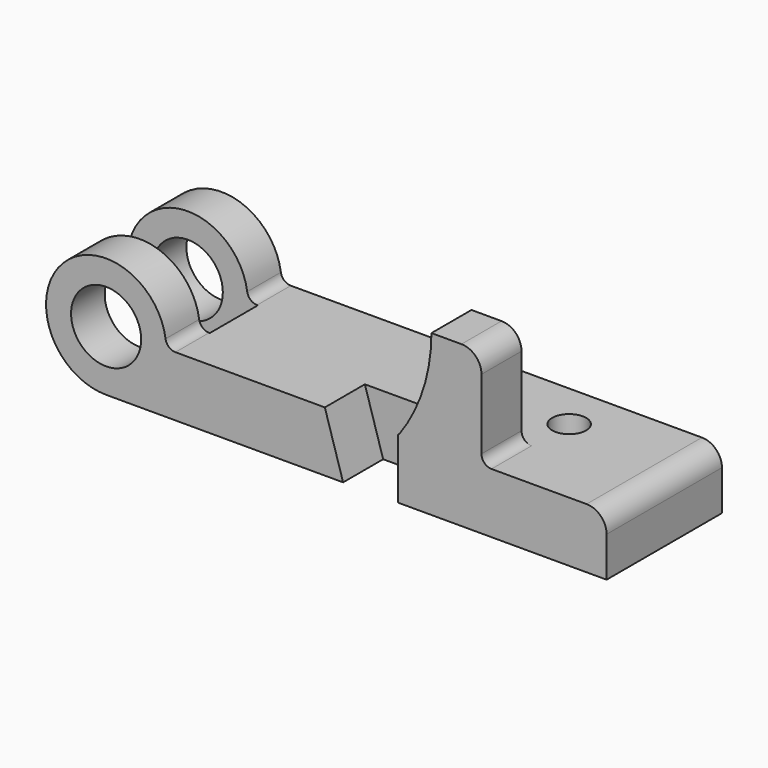
from build123d import *

# Parameters (mm, degrees)
F0_R      = 7
F1_DEPTH  = 14.4
F4_DEPTH  = 10
F7_DEPTH  = 10
F8_DEPTH  = 6
F9_R      = 3.4
F10_DEPTH = 25
F11_R     = 4
F12_R     = 2


with BuildPart() as f1:
    # F0 (on Front) → F1 (new body, symmetric)
    with BuildSketch(Plane.XZ):
        with BuildLine():
            Line((100, 0), (12, 0))
            ThreePointArc((12, 0), (-8.4852813742, 8.4852813742), (0, -12))
            Line((0, -12), (100, -12))
            Line((100, -12), (100, 0))
        make_face()
        Circle(F0_R, mode=Mode.SUBTRACT)
    extrude(amount=F1_DEPTH, both=True)

    # F3 (on face) → F4 (join)
    with BuildSketch(Plane.XZ.offset(14.4)):
        with BuildLine():
            Line((65, 0), (75, 0))
            Line((75, 0), (75, 20))
            Line((75, 20), (65, 20))
            ThreePointArc((65, 20), (63.3288514808, 9.4820344172), (58.48, 0))
            Line((58.48, 0), (65, 0))
        make_face()
    extrude(amount=-F4_DEPTH)

    # F6 (on face) → F7 (cut)
    with BuildSketch(Plane.XZ.offset(14.4)):
        Polygon((58.3458282053, -12), (58.3458282053, 0), (43.7034219503, 0), (47.3529601204, -12), align=None)
    extrude(amount=-F7_DEPTH, mode=Mode.SUBTRACT)

    # F2 (on Front) → F8 (cut, symmetric)
    with BuildSketch(Plane.XZ):
        with BuildLine():
            Line((14, -12), (14, 0))
            Line((14, 0), (12, 0))
            ThreePointArc((12, 0), (-8.4852813742, 8.4852813742), (0, -12))
            Line((0, -12), (14, -12))
        make_face()
    extrude(amount=F8_DEPTH, both=True, mode=Mode.SUBTRACT)

    # F9 (on face) → F10 (cut)
    with BuildSketch(Plane.XY):
        with Locations((77, 5)):
            Circle(F9_R)
    extrude(amount=-F10_DEPTH, mode=Mode.SUBTRACT)

    # F11
    f11_edges = [f1.edges().sort_by_distance(p)[0] for p in [
        (100, 0, 0),
        (75, -9.4, 20),
    ]]
    fillet(f11_edges, radius=F11_R)

    # F12
    f12_edges = [f1.edges().sort_by_distance(p)[0] for p in [
        (75, -9.4, 0),
        (12, 10.2, 0),
        (12, -10.2, 0),
    ]]
    fillet(f12_edges, radius=F12_R)


solid = f1.part
